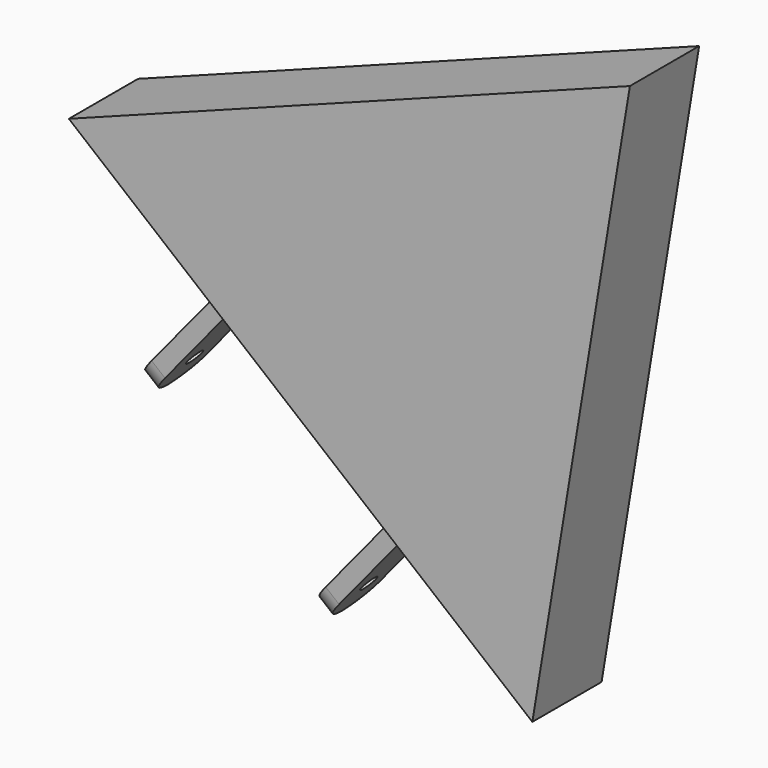
from build123d import *

# Parameters (mm, degrees)
F1_DEPTH    = 12.7
F2_W        = 2.54
F2_H        = 7.62
F3_DEPTH    = 20.32
F4_R        = 1.27
F5_DEPTH    = 25.4
F6_R        = 1.27
F7_DEPTH    = 25.4
F8_T1_DEPTH = 24.0023585695
F8_T3_DEPTH = 24.0023585695
F8_T5_DEPTH = 24.0023585695
F8_T7_DEPTH = 24.0023585695


# Not quite as in the source:
# - a fillet or chamfer that OpenCascade refuses, or shapes differently, is made with other operations: its cross-section is extruded or revolved along the edge and cut away or added


with BuildPart() as f1:
    # F0 (on Front) → F1 (new body)
    with BuildSketch(Plane.XZ):
        Polygon((32.2204480681, 39.2744538637), (-50.1228987998, 8.2664996165), (17.9024507316, -47.5409534801), align=None)
    extrude(amount=F1_DEPTH)

    # F2 (on face) → F3 (join)
    with BuildSketch(Plane(origin=(-16.1102240341, 0, -19.6372269318), x_dir=(0.7731191705, 0, -0.6342607887), z_dir=(-0.6342607887, 0, -0.7731191705))):
        with Locations((-16.51, 6.3304389822)):
            Rectangle(F2_W, F2_H)
        with Locations((16.51, 6.3037265553)):
            Rectangle(F2_W, F2_H)
    extrude(amount=F3_DEPTH)

    # F4 (on face) → F5 (cut)
    with BuildSketch(Plane(origin=(-13.7460588523, 0, 11.2771568238), x_dir=(0, -1, 0), z_dir=(-0.7731191705, 0, 0.6342607887))):
        with Locations((6.3304389822, -39.37)):
            Circle(F4_R)
    extrude(amount=-F5_DEPTH, mode=Mode.SUBTRACT)

    # F6 (on face) → F7 (cut)
    with BuildSketch(Plane(origin=(11.7823361591, 0, -9.6661344204), x_dir=(0, -1, 0), z_dir=(-0.7731191705, 0, 0.6342607887))):
        with Locations((6.3037265553, -39.37)):
            Circle(F6_R)
    extrude(amount=-F7_DEPTH, mode=Mode.SUBTRACT)

    # F8: fillet of radius 4.2924717139 on 4 edges, made by hand

    # F8_s2 → F8_t1 (cut)
    with BuildSketch(Plane(origin=(-22.0425392799, 0, 18.0835230611), x_dir=(0, 1, 0), z_dir=(0.7731191705, 0, -0.6342607887))):
        with BuildLine():
            ThreePointArc((-2.5204389822, -41.4275282861), (-3.7776748391, -44.4627641431), (-6.8129106961, -45.72))
            Line((-6.8129106961, -45.72), (-2.5204389822, -45.72))
            Line((-2.5204389822, -45.72), (-2.5204389822, -41.4275282861))
        make_face()
    extrude(amount=F8_T1_DEPTH, mode=Mode.SUBTRACT)

    # F8_s4 → F8_t3 (cut)
    with BuildSketch(Plane(origin=(-3.4858557315, 0, 2.8597681832), x_dir=(0, 1, 0), z_dir=(-0.7731191705, 0, 0.6342607887))):
        with BuildLine():
            ThreePointArc((-10.1404389822, 41.4275282861), (-8.8832031252, 44.4627641431), (-5.8479672683, 45.72))
            Line((-5.8479672683, 45.72), (-10.1404389822, 45.72))
            Line((-10.1404389822, 45.72), (-10.1404389822, 41.4275282861))
        make_face()
    extrude(amount=F8_T3_DEPTH, mode=Mode.SUBTRACT)

    # F8_s6 → F8_t5 (cut)
    with BuildSketch(Plane(origin=(3.4858557315, 0, -2.8597681832), x_dir=(0, 1, 0), z_dir=(0.7731191705, 0, -0.6342607887))):
        with BuildLine():
            ThreePointArc((-2.4937265553, -41.4275282861), (-3.7509624122, -44.4627641431), (-6.7861982692, -45.72))
            Line((-6.7861982692, -45.72), (-2.4937265553, -45.72))
            Line((-2.4937265553, -45.72), (-2.4937265553, -41.4275282861))
        make_face()
    extrude(amount=F8_T5_DEPTH, mode=Mode.SUBTRACT)

    # F8_s8 → F8_t7 (cut)
    with BuildSketch(Plane(origin=(22.0425392799, 0, -18.0835230611), x_dir=(0, 1, 0), z_dir=(-0.7731191705, 0, 0.6342607887))):
        with BuildLine():
            ThreePointArc((-10.1137265553, 41.4275282861), (-8.8564906983, 44.4627641431), (-5.8212548414, 45.72))
            Line((-5.8212548414, 45.72), (-10.1137265553, 45.72))
            Line((-10.1137265553, 45.72), (-10.1137265553, 41.4275282861))
        make_face()
    extrude(amount=F8_T7_DEPTH, mode=Mode.SUBTRACT)


solid = f1.part
